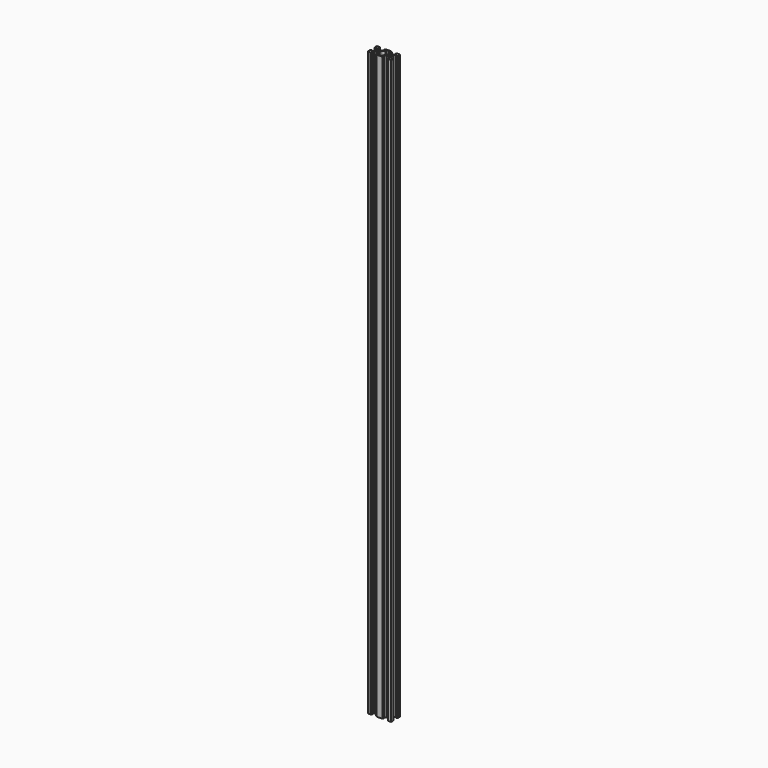
from build123d import *

# Parameters (mm, degrees)
F0_R     = 2.1
F1_DEPTH = 1000


# Not quite as in the source:
# - ends of sketch curves that miss each other by under 0.0002 mm in the source are joined


with BuildPart() as f1:
    # F0 (on Top) → F1 (new body)
    with BuildSketch(Plane.XY):
        with BuildLine():
            Line((-2.860219, 3.085333), (-2.860219, 5.198566))
            ThreePointArc((-2.860219, 5.198566), (-2.7720364303, 5.4101211696), (-2.56022, 5.497674))
            Line((-2.56022, 5.497674), (-1.22022, 5.497674))
            Line((-1.22022, 5.497674), (1.349586, 2.927868))
            ThreePointArc((1.349586, 2.927868), (1.4146178598, 2.8305410297), (1.437454, 2.715736))
            Line((1.437454, 2.715736), (1.437454, 0.1))
            Line((1.437454, 0.1), (1.637454, 0))
            Line((1.637454, 0), (1.437454, -0.1))
            Line((1.437454, -0.1), (1.437454, -2.715736))
            ThreePointArc((1.437454, -2.715736), (1.4146178598, -2.8305410297), (1.3495860344, -2.9278680344))
            Line((1.3495860344, -2.9278680344), (-1.22022, -5.497674))
            Line((-1.22022, -5.497674), (-2.56022, -5.497674))
            ThreePointArc((-2.56022, -5.497674), (-2.7720364303, -5.4101211696), (-2.8602186739, -5.198565999))
            Line((-2.8602186739, -5.198565999), (-2.860219, -3.085333))
            Line((-2.860219, -3.085333), (-4.661886, -4.887))
            Line((-4.661886, -4.887), (-4.661886, -9.6))
            ThreePointArc((-4.661886, -9.6), (-4.5447287125, -9.8828427125), (-4.261886, -10))
            Line((-4.261886, -10), (0.451114, -10))
            Line((0.451114, -10), (2.252781, -8.198333))
            Line((2.252781, -8.198333), (0.139548, -8.198333))
            ThreePointArc((0.139548, -8.198333), (-0.0720071696, -8.1101504303), (-0.15956, -7.898334))
            Line((-0.15956, -7.898334), (-0.15956, -6.558334))
            Line((-0.15956, -6.558334), (2.410246, -3.988528))
            ThreePointArc((2.410246, -3.988528), (2.5075729703, -3.9234961402), (2.622378, -3.90066))
            Line((2.622378, -3.90066), (5.238114, -3.90066))
            Line((5.238114, -3.90066), (5.338114, -3.70066))
            Line((5.338114, -3.70066), (5.438114, -3.90066))
            Line((5.438114, -3.90066), (8.05385, -3.90066))
            ThreePointArc((8.05385, -3.90066), (8.1686550297, -3.9234961402), (8.2659820344, -3.9885279656))
            Line((8.2659820344, -3.9885279656), (10.835788, -6.558334))
            Line((10.835788, -6.558334), (10.835788, -7.898334))
            ThreePointArc((10.835788, -7.898334), (10.7482351696, -8.1101504303), (10.536679999, -8.1983326739))
            Line((10.536679999, -8.1983326739), (8.423447, -8.198333))
            Line((8.423447, -8.198333), (10.225114, -10))
            Line((10.225114, -10), (20.451114, -10))
            Line((20.451114, -10), (22.252781, -8.198333))
            Line((22.252781, -8.198333), (20.139548, -8.198333))
            ThreePointArc((20.139548, -8.198333), (19.9279928304, -8.1101504303), (19.84044, -7.898334))
            Line((19.84044, -7.898334), (19.84044, -6.558334))
            Line((19.84044, -6.558334), (22.410246, -3.988528))
            ThreePointArc((22.410246, -3.988528), (22.5075729703, -3.9234961402), (22.622378, -3.90066))
            Line((22.622378, -3.90066), (25.238114, -3.90066))
            Line((25.238114, -3.90066), (25.338114, -3.70066))
            Line((25.338114, -3.70066), (25.438114, -3.90066))
            Line((25.438114, -3.90066), (28.05385, -3.90066))
            ThreePointArc((28.05385, -3.90066), (28.1686550297, -3.9234961402), (28.2659820344, -3.9885279656))
            Line((28.2659820344, -3.9885279656), (30.835788, -6.558334))
            Line((30.835788, -6.558334), (30.835788, -7.898334))
            ThreePointArc((30.835788, -7.898334), (30.7482351696, -8.1101504303), (30.536679999, -8.1983326739))
            Line((30.536679999, -8.1983326739), (28.423447, -8.198333))
            Line((28.423447, -8.198333), (30.225114, -10))
            Line((30.225114, -10), (34.938114, -10))
            ThreePointArc((34.938114, -10), (35.2209567125, -9.8828427125), (35.338114, -9.6))
            Line((35.338114, -9.6), (35.338114, -4.887))
            Line((35.338114, -4.887), (33.536447, -3.085333))
            Line((33.536447, -3.085333), (33.536447, -5.198566))
            ThreePointArc((33.536447, -5.198566), (33.4482644303, -5.4101211696), (33.236448, -5.497674))
            Line((33.236448, -5.497674), (31.896448, -5.497674))
            Line((31.896448, -5.497674), (29.326642, -2.927868))
            ThreePointArc((29.326642, -2.927868), (29.2616101402, -2.8305410297), (29.238774, -2.715736))
            Line((29.238774, -2.715736), (29.238774, -0.1))
            Line((29.238774, -0.1), (29.038774, 0))
            Line((29.038774, 0), (29.238774, 0.1))
            Line((29.238774, 0.1), (29.238774, 2.715736))
            ThreePointArc((29.238774, 2.715736), (29.2616101402, 2.8305410297), (29.3266419656, 2.9278680344))
            Line((29.3266419656, 2.9278680344), (31.896448, 5.497674))
            Line((31.896448, 5.497674), (33.236448, 5.497674))
            ThreePointArc((33.236448, 5.497674), (33.4482644303, 5.4101211696), (33.5364466739, 5.198565999))
            Line((33.5364466739, 5.198565999), (33.536447, 3.085333))
            Line((33.536447, 3.085333), (35.338114, 4.887))
            Line((35.338114, 4.887), (35.338114, 9.6))
            ThreePointArc((35.338114, 9.6), (35.2209567125, 9.8828427125), (34.938114, 10))
            Line((34.938114, 10), (30.225114, 10))
            Line((30.225114, 10), (28.423447, 8.198333))
            Line((28.423447, 8.198333), (30.53668, 8.198333))
            ThreePointArc((30.53668, 8.198333), (30.7482351696, 8.1101504303), (30.835788, 7.898334))
            Line((30.835788, 7.898334), (30.835788, 6.558334))
            Line((30.835788, 6.558334), (28.265982, 3.988528))
            ThreePointArc((28.265982, 3.988528), (28.1686550297, 3.9234961402), (28.05385, 3.90066))
            Line((28.05385, 3.90066), (25.438114, 3.90066))
            Line((25.438114, 3.90066), (25.338114, 3.70066))
            Line((25.338114, 3.70066), (25.238114, 3.90066))
            Line((25.238114, 3.90066), (22.622378, 3.90066))
            ThreePointArc((22.622378, 3.90066), (22.5075729703, 3.9234961402), (22.4102459656, 3.9885279656))
            Line((22.4102459656, 3.9885279656), (19.84044, 6.558334))
            Line((19.84044, 6.558334), (19.84044, 7.898334))
            ThreePointArc((19.84044, 7.898334), (19.9279928304, 8.1101504303), (20.139548001, 8.1983326739))
            Line((20.139548001, 8.1983326739), (22.252781, 8.198333))
            Line((22.252781, 8.198333), (20.451114, 10))
            Line((20.451114, 10), (10.225114, 10))
            Line((10.225114, 10), (8.423447, 8.198333))
            Line((8.423447, 8.198333), (10.53668, 8.198333))
            ThreePointArc((10.53668, 8.198333), (10.7482351696, 8.1101504303), (10.835788, 7.898334))
            Line((10.835788, 7.898334), (10.835788, 6.558334))
            Line((10.835788, 6.558334), (8.265982, 3.988528))
            ThreePointArc((8.265982, 3.988528), (8.1686550297, 3.9234961402), (8.05385, 3.90066))
            Line((8.05385, 3.90066), (5.438114, 3.90066))
            Line((5.438114, 3.90066), (5.338114, 3.70066))
            Line((5.338114, 3.70066), (5.238114, 3.90066))
            Line((5.238114, 3.90066), (2.622378, 3.90066))
            ThreePointArc((2.622378, 3.90066), (2.5075729703, 3.9234961402), (2.4102459656, 3.9885279656))
            Line((2.4102459656, 3.9885279656), (-0.15956, 6.558334))
            Line((-0.15956, 6.558334), (-0.15956, 7.898334))
            ThreePointArc((-0.15956, 7.898334), (-0.0720071696, 8.1101504303), (0.139548001, 8.1983326739))
            Line((0.139548001, 8.1983326739), (2.252781, 8.198333))
            Line((2.252781, 8.198333), (0.451114, 10))
            Line((0.451114, 10), (-4.261886, 10))
            ThreePointArc((-4.261886, 10), (-4.5447287125, 9.8828427125), (-4.661886, 9.6))
            Line((-4.661886, 9.6), (-4.661886, 4.887))
            Line((-4.661886, 4.887), (-2.860219, 3.085333))
        make_face()
        with Locations((5.338114, 0)):
            Circle(F0_R, mode=Mode.SUBTRACT)
        Polygon((12.638114, 6.24), (12.638114, 8.2), (18.038114, 8.2), (18.038114, 6.24), (21.349586, 2.927868), (21.437454, 2.715736), (21.437454, 0.1), (21.637454, 0), (21.437454, -0.1), (21.437454, -2.715736), (21.267706, -3.009748), (18.038114, -6.24), (18.037784, -8.2), (12.638114, -8.2), (12.638444, -6.23967), (9.326642, -2.927868), (9.238774, -2.715736), (9.238774, -0.1), (9.038774, 0), (9.238774, 0.1), (9.238774, 2.715736), (9.326642, 2.927868), align=None, mode=Mode.SUBTRACT)
        with Locations((25.338114, 0)):
            Circle(F0_R, mode=Mode.SUBTRACT)
    extrude(amount=F1_DEPTH)


solid = f1.part
